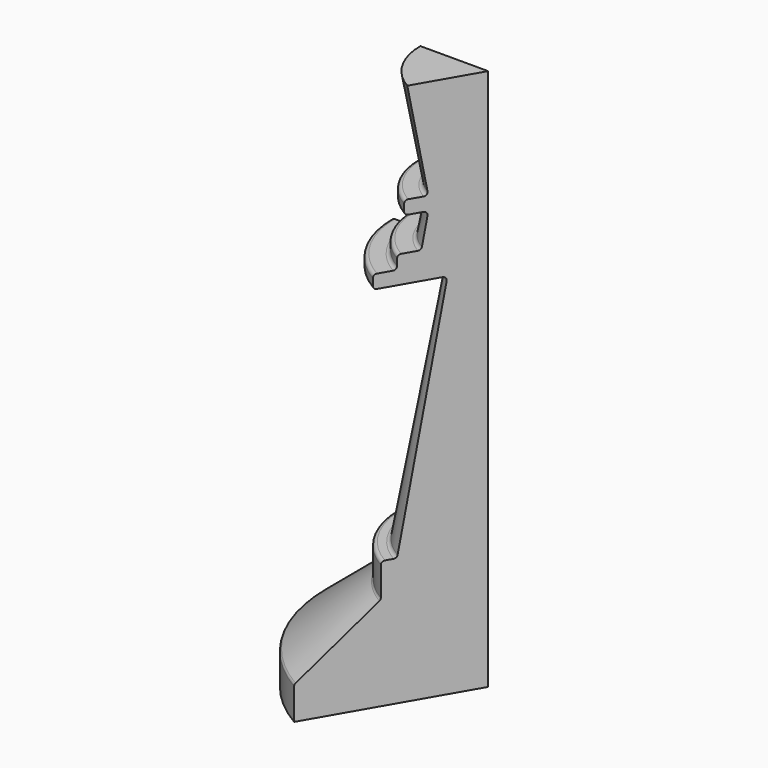
from build123d import *

# Parameters (mm, degrees)
F1_ANGLE = 60


# Not quite as in the source:
# - a feature of the source that left no trace in its solid (it failed there, or was rolled back) is left out


with BuildPart() as f1:
    # F0 (on Front) → F1 (revolve)
    with BuildSketch(Plane.XZ):
        with BuildLine():
            Line((-15.24, 0), (0, 0))
            Line((0, 0), (0, 50.8))
            Line((0, 50.8), (-6.35, 50.8))
            Line((-6.35, 50.8), (-4.7617064118, 41.792339449))
            ThreePointArc((-4.7617064118, 41.792339449), (-4.8311637627, 41.5331210865), (-5.0743828734, 41.4197061526))
            Line((-5.0743828734, 41.4197061526), (-6.2835011077, 41.4197061526))
            ThreePointArc((-6.2835011077, 41.4197061526), (-6.5080075107, 41.3267125556), (-6.6010011077, 41.1022061526))
            Line((-6.6010011077, 41.1022061526), (-6.6010011077, 40.4672061526))
            ThreePointArc((-6.6010011077, 40.4672061526), (-6.5080075107, 40.2426997495), (-6.2835011077, 40.1497061526))
            Line((-6.2835011077, 40.1497061526), (-5.0743828734, 40.1497061526))
            ThreePointArc((-5.0743828734, 40.1497061526), (-4.8311637627, 40.0362912186), (-4.7617064118, 39.7770728561))
            Line((-4.7617064118, 39.7770728561), (-5.2010717431, 37.2853082403))
            ThreePointArc((-5.2010717431, 37.2853082403), (-5.3096631386, 37.0972224261), (-5.5137482047, 37.0229415367))
            Line((-5.5137482047, 37.0229415367), (-6.8348340718, 37.0229415367))
            ThreePointArc((-6.8348340718, 37.0229415367), (-7.0593404748, 36.9299479398), (-7.1523340718, 36.7054415367))
            Line((-7.1523340718, 36.7054415367), (-7.1523340718, 36.0704415367))
            ThreePointArc((-7.1523340718, 36.0704415367), (-7.2453276688, 35.8459351337), (-7.4698340718, 35.7529415367))
            Line((-7.4698340718, 35.7529415367), (-8.7398340718, 35.7529415367))
            ThreePointArc((-8.7398340718, 35.7529415367), (-8.9643404748, 35.6599479398), (-9.0573340718, 35.4354415367))
            Line((-9.0573340718, 35.4354415367), (-9.0573340718, 34.8004415367))
            ThreePointArc((-9.0573340718, 34.8004415367), (-8.9643404748, 34.5759351337), (-8.7398340718, 34.4829415367))
            Line((-8.7398340718, 34.4829415367), (-3.5686493249, 34.4829415367))
            ThreePointArc((-3.5686493249, 34.4829415367), (-3.3254302142, 34.3695266028), (-3.2559728633, 34.1103082403))
            Line((-3.2559728633, 34.1103082403), (-7.113602572, 12.2326030065))
            ThreePointArc((-7.113602572, 12.2326030065), (-7.2221939675, 12.0445171922), (-7.4262790336, 11.9702363029))
            Line((-7.4262790336, 11.9702363029), (-8.1123649007, 11.9702363029))
            ThreePointArc((-8.1123649007, 11.9702363029), (-8.3368713037, 11.8772427059), (-8.4298649007, 11.6527363029))
            Line((-8.4298649007, 11.6527363029), (-8.4298649007, 8.9432889844))
            ThreePointArc((-8.4298649007, 8.9432889844), (-8.4596121783, 8.8091076862), (-8.5432798346, 8.7000698737))
            Line((-8.5432798346, 8.7000698737), (-15.1265850661, 3.176020882))
            ThreePointArc((-15.1265850661, 3.176020882), (-15.2102527224, 3.0669830694), (-15.24, 2.9328017713))
            Line((-15.24, 2.9328017713), (-15.24, 0))
        make_face()
    revolve(axis=Axis((0, 0, 25.4), (0, 0, 1)), revolution_arc=F1_ANGLE)


solid = f1.part
